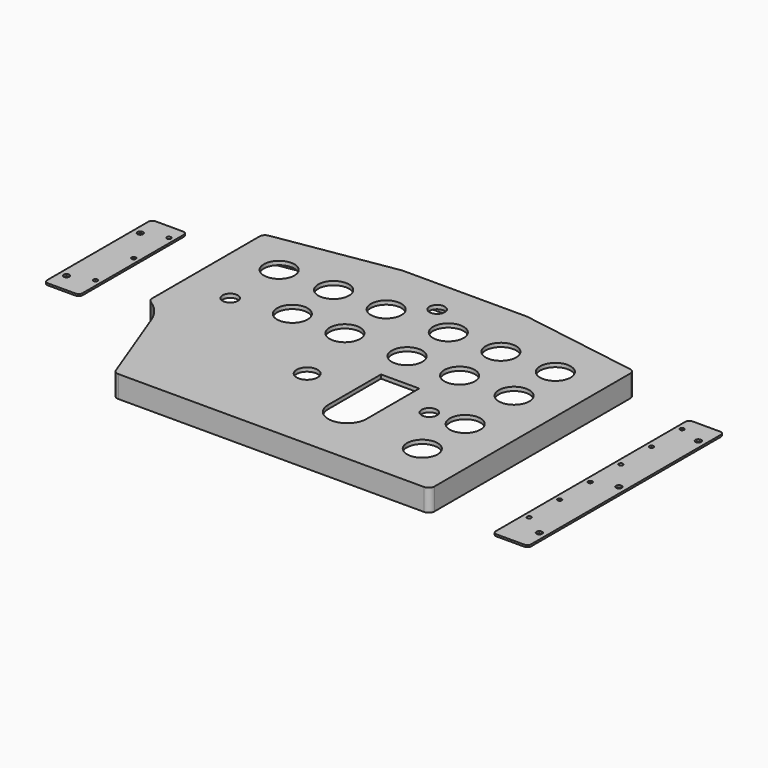
from build123d import *

# Parameters (mm, degrees)
F1_DEPTH  = 11.5
F2_T      = -2
F3_R      = 8
F3_R_2    = 5.5
F3_R_3    = 4
F4_DEPTH  = 5
F5_W      = 17.5
F5_H      = 70.271
F5_R      = 1.5
F5_R_2    = 1.1
F6_DEPTH  = 1
F7_W      = 17.5
F7_H      = 128.03771
F7_R      = 1.1
F7_R_2    = 1.5
F8_DEPTH  = 1
F9_DEPTH  = 1
F10_DEPTH = 1
F11_R     = 2
F11_2_R   = 2


# Not quite as in the source:
# - a feature names something its author has since deleted; it is built from what else it names


with BuildPart() as f1:
    # F0 (on Top) → F1 (new body)
    with BuildSketch(Plane.XY):
        with BuildLine():
            ThreePointArc((171.5266849444, -107.4031078396), (172.6273975977, -108.8098587101), (174.3326117763, -109.3416114362))
            Line((174.3326117763, -109.3416114362), (334.3326117763, -109.3416114362))
            ThreePointArc((334.3326117763, -109.3416114362), (336.4539321198, -108.4629317798), (337.3326117763, -106.3416114362))
            Line((337.3326117763, -106.3416114362), (337.3326117763, 21.6960972542))
            ThreePointArc((337.3326117763, 21.6960972542), (336.6166422945, 23.6411434212), (334.8104753818, 24.6577937907))
            Line((334.8104753818, 24.6577937907), (272.8326117763, 34.6577937907))
            Line((272.8326117763, 34.6577937907), (207.8326117763, 34.6577937907))
            Line((207.8326117763, 34.6577937907), (145.8547481708, 24.6577937907))
            ThreePointArc((145.8547481708, 24.6577937907), (144.048581258, 23.6411434212), (143.3326117763, 21.6960972542))
            Line((143.3326117763, 21.6960972542), (143.3326117763, -48.5747770261))
            ThreePointArc((143.3326117763, -48.5747770261), (143.7099796866, -50.0314173119), (144.7471457245, -51.1215980639))
            ThreePointArc((144.7471457245, -51.1215980639), (150.8507076214, -56.4737273832), (154.9176522246, -63.4993033507))
            Line((154.9176522246, -63.4993033507), (171.5266849444, -107.4031078396))
        make_face()
    extrude(amount=F1_DEPTH)

    # F2
    f2_openings = [f1.faces().sort_by_distance(p)[0] for p in [
        (243.718427, -37.163876, 0),
    ]]
    offset(amount=F2_T, openings=f2_openings)

    # F3 (on face) → F4 (cut)
    with BuildSketch(Plane.XY.offset(11.5)):
        with Locations((168.0826117763, 3.6573637907)):
            Circle(F3_R)
        with Locations((196.5826117763, 3.6573637907)):
            Circle(F3_R)
        with Locations((224.0826117763, 3.6573637907)):
            Circle(F3_R)
        with Locations((256.5826117763, 3.6573637907)):
            Circle(F3_R)
        with Locations((284.0826117763, 3.6573637907)):
            Circle(F3_R)
        with Locations((312.5826117763, 3.6573637907)):
            Circle(F3_R)
        with BuildLine():
            Line((278.3326103382, -42.5556362093), (258.3326103382, -42.5556362093))
            Line((258.3326103382, -42.5556362093), (258.3326103382, -77.0556362093))
            ThreePointArc((258.3326103382, -77.0556362093), (261.2615425264, -84.1267040211), (268.3326103382, -87.0556362093))
            ThreePointArc((268.3326103382, -87.0556362093), (275.4036781501, -84.1267040211), (278.3326103382, -77.0556362093))
            Line((278.3326103382, -77.0556362093), (278.3326103382, -42.5556362093))
        make_face()
        with Locations((312.5826117763, -55.3422062093)):
            Circle(F3_R)
        with Locations((312.5826117763, -83.3422062093)):
            Circle(F3_R)
        with Locations((234.3326103382, -60.8422062093)):
            Circle(F3_R_2)
        with Locations((294.8326117763, -56.5556362093)):
            Circle(F3_R_3)
        with Locations((240.3326117763, 16.6573637907)):
            Circle(F3_R_3)
        with Locations((168.0826117763, -28.3426362093)):
            Circle(F3_R_3)
        with Locations((196.5826117763, -23.3426362093)):
            Circle(F3_R)
        with Locations((224.0826117763, -23.3426362093)):
            Circle(F3_R)
        with Locations((256.5826117763, -23.3426362093)):
            Circle(F3_R)
        with Locations((284.0826117763, -23.3426362093)):
            Circle(F3_R)
        with Locations((312.5826117763, -23.3426362093)):
            Circle(F3_R)
    extrude(amount=-F4_DEPTH, mode=Mode.SUBTRACT)


with BuildPart() as f6:
    # F5 (on Top) → F6 (new body)
    with BuildSketch(Plane.XY):
        with Locations((95.8951199055, -13.7335582237)):
            Rectangle(F5_W, F5_H)
        with Locations((90.8951199055, -38.8689282237)):
            Circle(F5_R, mode=Mode.SUBTRACT)
        with Locations((102.6451199055, -34.5980582237)):
            Circle(F5_R_2, mode=Mode.SUBTRACT)
        with Locations((90.8951199055, 9.4019417763)):
            Circle(F5_R, mode=Mode.SUBTRACT)
        with Locations((102.6451199055, -9.5980582237)):
            Circle(F5_R_2, mode=Mode.SUBTRACT)
        with Locations((102.6451199055, 13.4019417763)):
            Circle(F5_R_2, mode=Mode.SUBTRACT)
    extrude(amount=F6_DEPTH)

    # F10 (add): a face of the model
    f10_faces = [f6.faces().sort_by_distance(p)[0] for p in [
        (104.6451199055, -13.7335582237, 0.5),
    ]]
    extrude(f10_faces, amount=F10_DEPTH)

    # F11#2
    f11_2_edges = [f6.edges().sort_by_distance(p)[0] for p in [
        (105.64512, -48.869058, 0.5),
        (87.14512, -48.869058, 0.5),
        (105.64512, 21.401942, 0.5),
        (87.14512, 21.401942, 0.5),
    ]]
    fillet(f11_2_edges, radius=F11_2_R)


with BuildPart() as f8:
    # F7 (on Top) → F8 (new body)
    with BuildSketch(Plane.XY):
        with Locations((378.7404644489, -43.7870440428)):
            Rectangle(F7_W, F7_H)
        with Locations((371.9904644489, -87.7681890428)):
            Circle(F7_R, mode=Mode.SUBTRACT)
        with Locations((371.9904644489, -67.7681890428)):
            Circle(F7_R, mode=Mode.SUBTRACT)
        with Locations((371.9904644489, -47.7681890428)):
            Circle(F7_R, mode=Mode.SUBTRACT)
        with Locations((383.7404644489, -95.8058990428)):
            Circle(F7_R_2, mode=Mode.SUBTRACT)
        with Locations((371.9904644489, -27.7681890428)):
            Circle(F7_R, mode=Mode.SUBTRACT)
        with Locations((371.9904644489, -7.7681890428)):
            Circle(F7_R, mode=Mode.SUBTRACT)
        with Locations((371.9904644489, 12.2318109572)):
            Circle(F7_R, mode=Mode.SUBTRACT)
        with Locations((383.7404644489, -43.7681890428)):
            Circle(F7_R_2, mode=Mode.SUBTRACT)
        with Locations((383.7404644489, 8.2318109572)):
            Circle(F7_R_2, mode=Mode.SUBTRACT)
    extrude(amount=F8_DEPTH)

    # F9 (add): a face of the model
    f9_faces = [f8.faces().sort_by_distance(p)[0] for p in [
        (369.9904644489, -43.7870440428, 0.5),
    ]]
    extrude(f9_faces, amount=F9_DEPTH)

    # F11
    f11_edges = [f8.edges().sort_by_distance(p)[0] for p in [
        (387.490464, 20.231811, 0.5),
        (368.990464, 20.231811, 0.5),
        (387.490464, -107.805899, 0.5),
        (368.990464, -107.805899, 0.5),
    ]]
    fillet(f11_edges, radius=F11_R)


solid = Compound([f1.part, f6.part, f8.part])
